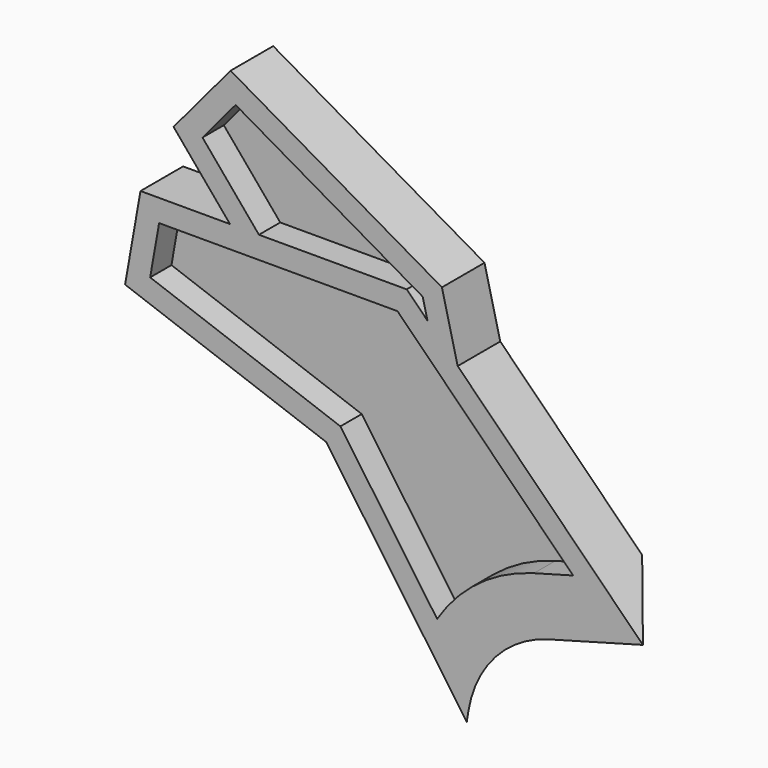
from build123d import *

# Parameters (mm, degrees)
F1_DEPTH    = 24
F2_R        = 50
F3_T1_DEPTH = 105.7731172378
F3_T3_DEPTH = 66.3378383392
F3_T6_ANGLE = 65.4740658064
F6_DEPTH    = 12
F8_DEPTH    = 12
F9_DEPTH    = 12
F11_DEPTH   = 12


# Not quite as in the source:
# - a fillet or chamfer that OpenCascade refuses, or shapes differently, is made with other operations: its cross-section is extruded or revolved along the edge and cut away or added


with BuildPart() as f1:
    # F0 (on Front) → F1 (new body)
    with BuildSketch(Plane.XZ):
        Polygon((-81.055521965, 64.9488791823), (-7.5541026236, 85.0398655279), (-114.0252747561, 191.5110376604), (-234.0252747561, 191.5110376604), (-240.9712018628, 152.1187275399), (-150.2916823338, 119.1140815738), (-86.9572677666, 28.6631636514), align=None)
    extrude(amount=F1_DEPTH)

    # F2
    f2_edges = [f1.edges().sort_by_distance(p)[0] for p in [
        (-81.055522, -12, 64.948879),
    ]]
    fillet(f2_edges, radius=F2_R)

    # F3: chamfer of 24 on 2 edges, made by hand

    # F3_s2 → F3_t1 (cut)
    with BuildSketch(Plane(origin=(-27.8938692058, 0, -7.6245513401), x_dir=(0, 1, 0), z_dir=(0.9646132681, 0, 0.2636688131))):
        Polygon((0, 108.0223638788), (-24, 84.0223638788), (0, 84.0223638788), align=None)
    extrude(amount=F3_T1_DEPTH, mode=Mode.SUBTRACT)

    # F3_s4 → F3_t3 (cut)
    with BuildSketch(Plane(origin=(-7.6076630021, 0, -46.7742096713), x_dir=(0, 1, 0), z_dir=(0.1605369785, 0, 0.9870298266))):
        Polygon((-24, 90.4309146097), (0, 114.4309146097), (0, 90.4309146097), align=None)
    extrude(amount=F3_T3_DEPTH, mode=Mode.SUBTRACT)

    # F3_s5 → F3_t6 (revolve, cut)
    with BuildSketch(Plane(origin=(3.0420131267, 0, 18.7032153992), x_dir=(0, 1, 0), z_dir=(-0.1605369785, 0, -0.9870298266))):
        Polygon((0, -114.4309146097), (-24, -90.4309146097), (0, -90.4309146097), align=None)
    revolve(axis=Axis((-36.8645055082, 0, 25.1938722697), (0, 1, 0)), revolution_arc=F3_T6_ANGLE, mode=Mode.SUBTRACT)

    # F5 (on face) → F6 (join)
    with BuildSketch(Plane(origin=(0, 0, 0), x_dir=(-1, 0, 0), z_dir=(0, 1, 0))):
        Polygon((84.0423926711, 139.9491429329), (163.5881303991, 155.6373062127), (219.1278844576, 221.8270076437), (193.4163800701, 252.4687853684), (98.1535856538, 197.4687853684), align=None)
    extrude(amount=-F6_DEPTH)

    # F7 (on face) → F8 (cut)
    with BuildSketch(Plane.XZ.offset(24)):
        with BuildLine():
            Line((-143.908641448, 127.432622412), (-100.3174393188, 65.1779339797))
            ThreePointArc((-100.3174393188, 65.1779339797), (-81.5137230154, 85.4553639206), (-56.6396664901, 97.5398673775))
            Line((-56.6396664901, 97.5398673775), (-39.014051648, 102.3576789286))
            Line((-39.014051648, 102.3576789286), (-118.1674103798, 181.5110376604))
            Line((-118.1674103798, 181.5110376604), (-225.6342784443, 181.5110376604))
            Line((-225.6342784443, 181.5110376604), (-229.6660431143, 158.6457639866))
            Line((-229.6660431143, 158.6457639866), (-143.908641448, 127.432622412))
        make_face()
    extrude(amount=-F8_DEPTH, mode=Mode.SUBTRACT)

    # F9 (add): a face of the model
    f9_faces = [f1.faces().sort_by_distance(p)[0] for p in [
        (-164.1324178165, -12, 212.498446066),
    ]]
    extrude(f9_faces, amount=F9_DEPTH)

    # F10 (on face) → F11 (cut)
    with BuildSketch(Plane.XZ.offset(24)):
        Polygon((-104.7010093218, 182.1867722261), (-106.848922609, 190.9420351164), (-191.149564101, 239.6130331747), (-206.0738115642, 221.8270076437), (-180.6356923325, 191.5110376604), (-114.0252747561, 191.5110376604), align=None)
    extrude(amount=-F11_DEPTH, mode=Mode.SUBTRACT)


solid = f1.part
